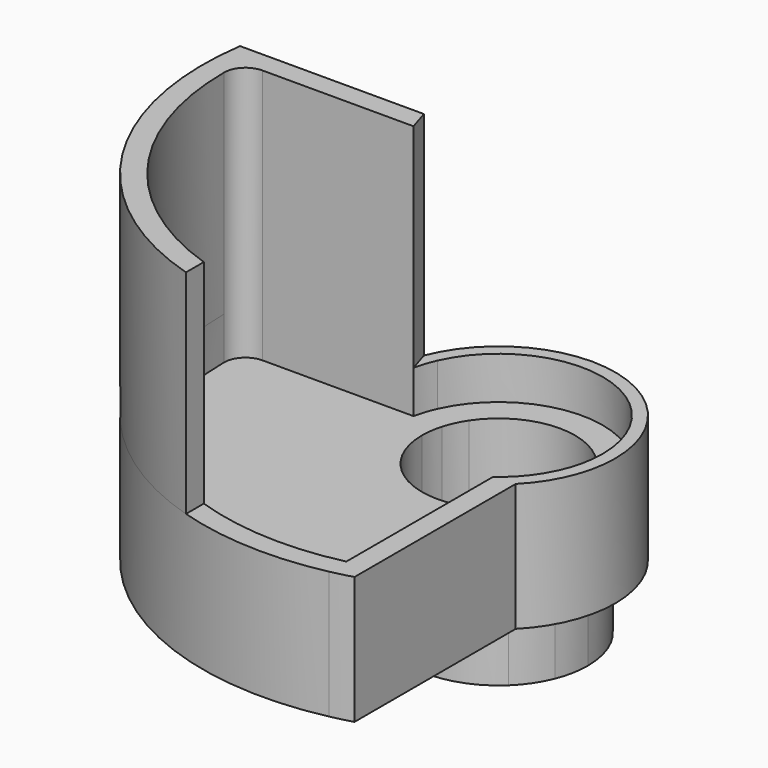
from build123d import *

# Parameters (mm, degrees)
F1_DEPTH    = 2
F2_DEPTH    = 3
F3_DEPTH    = 1.5
F5_DEPTH    = 5
F6_T1_DEPTH = 7.2509414233


# Not quite as in the source:
# - a fillet or chamfer that OpenCascade refuses, or shapes differently, is made with other operations: its cross-section is extruded or revolved along the edge and cut away or added
# - a feature names something its author has since deleted; it is built from what else it names


with BuildPart() as f1:
    # F0 (on Top) → F1 (new body)
    with BuildSketch(Plane.XY):
        with BuildLine():
            ThreePointArc((-2.398436991, 0.5), (-2.3309771289, 0.7543511281), (-2.2366269246, 1))
            Line((-2.2366269246, 1), (-2.556369496, 1))
            ThreePointArc((-2.556369496, 1), (-2.6395896521, 0.7533866658), (-2.6990785465, 0.5))
            Line((-2.6990785465, 0.5), (-2.398436991, 0.5))
        make_face()
        with BuildLine():
            ThreePointArc((-2.2366269246, 1), (0.5112553348, 2.3960630173), (2.45, 0))
            ThreePointArc((2.45, 0), (2.3216373532, -0.7826237921), (1.95, -1.4832396974))
            Line((1.95, -1.4832396974), (1.95, -1.9319743787))
            ThreePointArc((1.95, -1.9319743787), (2.5384813373, -1.0445752725), (2.745, 0))
            ThreePointArc((2.745, 0), (0.5088176164, 2.6974301906), (-2.556369496, 1))
            Line((-2.556369496, 1), (-2.2366269246, 1))
        make_face()
        with BuildLine():
            ThreePointArc((-2.6990785465, 0.5), (-2.6395896521, 0.7533866658), (-2.556369496, 1))
            Line((-2.556369496, 1), (-6.3720091023, 1))
            ThreePointArc((-6.3720091023, 1), (-6.4061799882, 0.7505717543), (-6.4305909526, 0.5))
            Line((-6.4305909526, 0.5), (-2.6990785465, 0.5))
        make_face()
        with BuildLine():
            ThreePointArc((-2.745, 0), (-2.7334955286, 0.2510521758), (-2.6990785465, 0.5))
            Line((-2.6990785465, 0.5), (-6.4305909526, 0.5))
            ThreePointArc((-6.4305909526, 0.5), (-6.4451459116, 0.2501882847), (-6.45, 0))
            Line((-6.45, 0), (-2.745, 0))
        make_face()
        with BuildLine():
            Line((1.45, -6.284902545), (1.45, -2.3307777672))
            ThreePointArc((1.45, -2.3307777672), (-1.3331869711, -2.399507762), (-2.745, 0))
            Line((-2.745, 0), (-6.45, 0))
            ThreePointArc((-6.45, 0), (-4.0155946011, -5.0475241456), (1.45, -6.284902545))
        make_face()
        with BuildLine():
            Line((1.45, -2.3307777672), (1.45, -1.9748417658))
            ThreePointArc((1.45, -1.9748417658), (-1.1067971811, -2.1857492994), (-2.45, 0))
            Line((-2.45, 0), (-2.745, 0))
            ThreePointArc((-2.745, 0), (-1.3331869711, -2.399507762), (1.45, -2.3307777672))
        make_face()
        with BuildLine():
            Line((1.95, -1.9319743787), (1.95, -1.4832396974))
            ThreePointArc((1.95, -1.4832396974), (1.7176781271, -1.7470208504), (1.45, -1.9748417658))
            Line((1.45, -1.9748417658), (1.45, -2.3307777672))
            ThreePointArc((1.45, -2.3307777672), (1.7116544732, -2.1459878761), (1.95, -1.9319743787))
        make_face()
        with BuildLine():
            Line((1.95, -6.1481704596), (1.95, -1.9319743787))
            ThreePointArc((1.95, -1.9319743787), (1.7116544732, -2.1459878761), (1.45, -2.3307777672))
            Line((1.45, -2.3307777672), (1.45, -6.284902545))
            ThreePointArc((1.45, -6.284902545), (1.7013741258, -6.2215613864), (1.95, -6.1481704596))
        make_face()
        with BuildLine():
            ThreePointArc((-6.4305909526, 0.5), (-6.4061799882, 0.7505717543), (-6.3720091023, 1))
            Line((-6.3720091023, 1), (-6.8776812953, 1))
            ThreePointArc((-6.8776812953, 1), (-6.9093605068, 0.7504914307), (-6.931991056, 0.5))
            Line((-6.931991056, 0.5), (-6.4305909526, 0.5))
        make_face()
        with BuildLine():
            Line((1.95, -6.6708320321), (1.95, -6.1481704596))
            ThreePointArc((1.95, -6.1481704596), (1.7013741258, -6.2215613864), (1.45, -6.284902545))
            Line((1.45, -6.284902545), (1.45, -6.7970581872))
            ThreePointArc((1.45, -6.7970581872), (1.7011711438, -6.7385841791), (1.95, -6.6708320321))
        make_face()
        with BuildLine():
            Line((1.45, -6.7970581872), (1.45, -6.284902545))
            ThreePointArc((1.45, -6.284902545), (-4.0155946011, -5.0475241456), (-6.45, 0))
            Line((-6.45, 0), (-6.95, 0))
            ThreePointArc((-6.95, 0), (-4.3717845327, -5.4027770637), (1.45, -6.7970581872))
        make_face()
        with BuildLine():
            ThreePointArc((-6.45, 0), (-6.4451459116, 0.2501882847), (-6.4305909526, 0.5))
            Line((-6.4305909526, 0.5), (-6.931991056, 0.5))
            ThreePointArc((-6.931991056, 0.5), (-6.9454963048, 0.2501621085), (-6.95, 0))
            Line((-6.95, 0), (-6.45, 0))
        make_face()
        with BuildLine():
            ThreePointArc((-2.45, 0), (-2.4370751556, 0.2513258562), (-2.398436991, 0.5))
            Line((-2.398436991, 0.5), (-2.6990785465, 0.5))
            ThreePointArc((-2.6990785465, 0.5), (-2.7334955286, 0.2510521758), (-2.745, 0))
            Line((-2.745, 0), (-2.45, 0))
        make_face()
        with BuildLine():
            ThreePointArc((-2.45, 0), (-1.1067971811, -2.1857492994), (1.45, -1.9748417658))
            Line((1.45, -1.9748417658), (1.45, -1.5190457531))
            ThreePointArc((1.45, -1.5190457531), (-0.8261355821, -1.9306734576), (-2.1, 0))
            Line((-2.1, 0), (-2.45, 0))
        make_face()
        with BuildLine():
            ThreePointArc((-2.1, 0), (-0.8261355821, -1.9306734576), (1.45, -1.5190457531))
            Line((1.45, -1.5190457531), (1.45, -1.0665364504))
            ThreePointArc((1.45, -1.0665364504), (-0.561248608, -1.7102631376), (-1.8, 0))
            Line((-1.8, 0), (-2.1, 0))
        make_face()
        with BuildLine():
            Line((-2.0396078054, 0.5), (-2.398436991, 0.5))
            ThreePointArc((-2.398436991, 0.5), (-2.4370751556, 0.2513258562), (-2.45, 0))
            Line((-2.45, 0), (-2.1, 0))
            ThreePointArc((-2.1, 0), (-2.0848472835, 0.2518170056), (-2.0396078054, 0.5))
        make_face()
        with BuildLine():
            Line((-1.8466185313, 1), (-2.2366269246, 1))
            ThreePointArc((-2.2366269246, 1), (-2.3309771289, 0.7543511281), (-2.398436991, 0.5))
            Line((-2.398436991, 0.5), (-2.0396078054, 0.5))
            ThreePointArc((-2.0396078054, 0.5), (-1.9591295988, 0.7561819986), (-1.8466185313, 1))
        make_face()
        with BuildLine():
            Line((2.1, 0), (2.45, 0))
            ThreePointArc((2.45, 0), (0.5112553348, 2.3960630173), (-2.2366269246, 1))
            Line((-2.2366269246, 1), (-1.8466185313, 1))
            ThreePointArc((-1.8466185313, 1), (0.5158008745, 2.0356692899), (2.1, 0))
        make_face()
        with BuildLine():
            Line((-1.7291616466, 0.5), (-2.0396078054, 0.5))
            ThreePointArc((-2.0396078054, 0.5), (-2.0848472835, 0.2518170056), (-2.1, 0))
            Line((-2.1, 0), (-1.8, 0))
            ThreePointArc((-1.8, 0), (-1.7822024245, 0.2524965704), (-1.7291616466, 0.5))
        make_face()
        with BuildLine():
            Line((-1.4966629547, 1), (-1.8466185313, 1))
            ThreePointArc((-1.8466185313, 1), (-1.9591295988, 0.7561819986), (-2.0396078054, 0.5))
            Line((-2.0396078054, 0.5), (-1.7291616466, 0.5))
            ThreePointArc((-1.7291616466, 0.5), (-1.6321721997, 0.7589558027), (-1.4966629547, 1))
        make_face()
        with BuildLine():
            Line((1.95, 0), (2.1, 0))
            ThreePointArc((2.1, 0), (0.5158008745, 2.0356692899), (-1.8466185313, 1))
            Line((-1.8466185313, 1), (-1.4966629547, 1))
            ThreePointArc((-1.4966629547, 1), (0.522497216, 1.722497216), (1.8, 0))
            Line((1.8, 0), (1.95, 0))
        make_face()
        with BuildLine():
            ThreePointArc((1.45, -1.5190457531), (1.739758749, -1.176112025), (1.95, -0.7794228634))
            Line((1.95, -0.7794228634), (1.95, 0))
            Line((1.95, 0), (1.8, 0))
            ThreePointArc((1.8, 0), (1.7102631376, -0.561248608), (1.45, -1.0665364504))
            Line((1.45, -1.0665364504), (1.45, -1.5190457531))
        make_face()
        with BuildLine():
            ThreePointArc((1.45, -1.9748417658), (1.7176781271, -1.7470208504), (1.95, -1.4832396974))
            Line((1.95, -1.4832396974), (1.95, -0.7794228634))
            ThreePointArc((1.95, -0.7794228634), (1.739758749, -1.176112025), (1.45, -1.5190457531))
            Line((1.45, -1.5190457531), (1.45, -1.9748417658))
        make_face()
        with BuildLine():
            ThreePointArc((1.95, -0.7794228634), (2.0621590627, -0.3968626967), (2.1, 0))
            Line((2.1, 0), (1.95, 0))
            Line((1.95, 0), (1.95, -0.7794228634))
        make_face()
        with BuildLine():
            ThreePointArc((1.95, -1.4832396974), (2.3216373532, -0.7826237921), (2.45, 0))
            Line((2.45, 0), (2.1, 0))
            ThreePointArc((2.1, 0), (2.0621590627, -0.3968626967), (1.95, -0.7794228634))
            Line((1.95, -0.7794228634), (1.95, -1.4832396974))
        make_face()
    extrude(amount=F1_DEPTH)

    # F0 (on Top) → F2 (join)
    with BuildSketch(Plane.XY):
        with BuildLine():
            ThreePointArc((-6.4305909526, 0.5), (-6.4061799882, 0.7505717543), (-6.3720091023, 1))
            Line((-6.3720091023, 1), (-6.8776812953, 1))
            ThreePointArc((-6.8776812953, 1), (-6.9093605068, 0.7504914307), (-6.931991056, 0.5))
            Line((-6.931991056, 0.5), (-6.4305909526, 0.5))
        make_face()
        with BuildLine():
            ThreePointArc((-2.6990785465, 0.5), (-2.6395896521, 0.7533866658), (-2.556369496, 1))
            Line((-2.556369496, 1), (-6.3720091023, 1))
            ThreePointArc((-6.3720091023, 1), (-6.4061799882, 0.7505717543), (-6.4305909526, 0.5))
            Line((-6.4305909526, 0.5), (-2.6990785465, 0.5))
        make_face()
        with BuildLine():
            ThreePointArc((-2.398436991, 0.5), (-2.3309771289, 0.7543511281), (-2.2366269246, 1))
            Line((-2.2366269246, 1), (-2.556369496, 1))
            ThreePointArc((-2.556369496, 1), (-2.6395896521, 0.7533866658), (-2.6990785465, 0.5))
            Line((-2.6990785465, 0.5), (-2.398436991, 0.5))
        make_face()
        with BuildLine():
            ThreePointArc((-2.2366269246, 1), (0.5112553348, 2.3960630173), (2.45, 0))
            ThreePointArc((2.45, 0), (2.3216373532, -0.7826237921), (1.95, -1.4832396974))
            Line((1.95, -1.4832396974), (1.95, -1.9319743787))
            ThreePointArc((1.95, -1.9319743787), (2.5384813373, -1.0445752725), (2.745, 0))
            ThreePointArc((2.745, 0), (0.5088176164, 2.6974301906), (-2.556369496, 1))
            Line((-2.556369496, 1), (-2.2366269246, 1))
        make_face()
        with BuildLine():
            Line((1.95, -1.9319743787), (1.95, -1.4832396974))
            ThreePointArc((1.95, -1.4832396974), (1.7176781271, -1.7470208504), (1.45, -1.9748417658))
            Line((1.45, -1.9748417658), (1.45, -2.3307777672))
            ThreePointArc((1.45, -2.3307777672), (1.7116544732, -2.1459878761), (1.95, -1.9319743787))
        make_face()
        with BuildLine():
            Line((1.95, -6.1481704596), (1.95, -1.9319743787))
            ThreePointArc((1.95, -1.9319743787), (1.7116544732, -2.1459878761), (1.45, -2.3307777672))
            Line((1.45, -2.3307777672), (1.45, -6.284902545))
            ThreePointArc((1.45, -6.284902545), (1.7013741258, -6.2215613864), (1.95, -6.1481704596))
        make_face()
        with BuildLine():
            Line((1.95, -6.6708320321), (1.95, -6.1481704596))
            ThreePointArc((1.95, -6.1481704596), (1.7013741258, -6.2215613864), (1.45, -6.284902545))
            Line((1.45, -6.284902545), (1.45, -6.7970581872))
            ThreePointArc((1.45, -6.7970581872), (1.7011711438, -6.7385841791), (1.95, -6.6708320321))
        make_face()
        with BuildLine():
            Line((1.45, -6.7970581872), (1.45, -6.284902545))
            ThreePointArc((1.45, -6.284902545), (-4.0155946011, -5.0475241456), (-6.45, 0))
            Line((-6.45, 0), (-6.95, 0))
            ThreePointArc((-6.95, 0), (-4.3717845327, -5.4027770637), (1.45, -6.7970581872))
        make_face()
        with BuildLine():
            ThreePointArc((-6.45, 0), (-6.4451459116, 0.2501882847), (-6.4305909526, 0.5))
            Line((-6.4305909526, 0.5), (-6.931991056, 0.5))
            ThreePointArc((-6.931991056, 0.5), (-6.9454963048, 0.2501621085), (-6.95, 0))
            Line((-6.95, 0), (-6.45, 0))
        make_face()
    extrude(amount=F2_DEPTH)

    # F0 (on Top) → F3 (join)
    with BuildSketch(Plane.XY):
        with BuildLine():
            Line((1.95, 0), (2.1, 0))
            ThreePointArc((2.1, 0), (0.5158008745, 2.0356692899), (-1.8466185313, 1))
            Line((-1.8466185313, 1), (-1.4966629547, 1))
            ThreePointArc((-1.4966629547, 1), (0.522497216, 1.722497216), (1.8, 0))
            Line((1.8, 0), (1.95, 0))
        make_face()
        with BuildLine():
            Line((-1.4966629547, 1), (-1.8466185313, 1))
            ThreePointArc((-1.8466185313, 1), (-1.9591295988, 0.7561819986), (-2.0396078054, 0.5))
            Line((-2.0396078054, 0.5), (-1.7291616466, 0.5))
            ThreePointArc((-1.7291616466, 0.5), (-1.6321721997, 0.7589558027), (-1.4966629547, 1))
        make_face()
        with BuildLine():
            Line((-1.7291616466, 0.5), (-2.0396078054, 0.5))
            ThreePointArc((-2.0396078054, 0.5), (-2.0848472835, 0.2518170056), (-2.1, 0))
            Line((-2.1, 0), (-1.8, 0))
            ThreePointArc((-1.8, 0), (-1.7822024245, 0.2524965704), (-1.7291616466, 0.5))
        make_face()
        with BuildLine():
            ThreePointArc((-2.1, 0), (-0.8261355821, -1.9306734576), (1.45, -1.5190457531))
            Line((1.45, -1.5190457531), (1.45, -1.0665364504))
            ThreePointArc((1.45, -1.0665364504), (-0.561248608, -1.7102631376), (-1.8, 0))
            Line((-1.8, 0), (-2.1, 0))
        make_face()
        with BuildLine():
            ThreePointArc((1.45, -1.5190457531), (1.739758749, -1.176112025), (1.95, -0.7794228634))
            Line((1.95, -0.7794228634), (1.95, 0))
            Line((1.95, 0), (1.8, 0))
            ThreePointArc((1.8, 0), (1.7102631376, -0.561248608), (1.45, -1.0665364504))
            Line((1.45, -1.0665364504), (1.45, -1.5190457531))
        make_face()
        with BuildLine():
            ThreePointArc((1.95, -0.7794228634), (2.0621590627, -0.3968626967), (2.1, 0))
            Line((2.1, 0), (1.95, 0))
            Line((1.95, 0), (1.95, -0.7794228634))
        make_face()
    extrude(amount=-F3_DEPTH)

    # F4 (on face) → F5 (join)
    with BuildSketch(Plane.XY.offset(3)):
        with BuildLine():
            Line((-2.398436991, 0.5), (-2.556369496, 1))
            Line((-2.556369496, 1), (-6.8776812953, 1))
            ThreePointArc((-6.8776812953, 1), (-5.8706460858, -3.7199481898), (-2.0327166243, -6.6460938246))
            Line((-2.0327166243, -6.6460938246), (-2.0327166243, -6.1213203743))
            ThreePointArc((-2.0327166243, -6.1213203743), (-5.3728358118, -3.5686321385), (-6.4305909526, 0.5))
            Line((-6.4305909526, 0.5), (-2.398436991, 0.5))
        make_face()
    extrude(amount=F5_DEPTH)

    # F6: fillet of radius 0.5 on 1 edges, made by hand

    # F6_s2 → F6_t1 (join)
    with BuildSketch(Plane.XY.offset(0.7490585767)):
        with BuildLine():
            ThreePointArc((-5.95, 0.5), (-6.3035533906, 0.3535533906), (-6.45, 0))
            ThreePointArc((-6.45, 0), (-6.4451459116, 0.2501882847), (-6.4305909526, 0.5))
            Line((-6.4305909526, 0.5), (-5.95, 0.5))
        make_face()
    extrude(amount=F6_T1_DEPTH)


solid = f1.part
